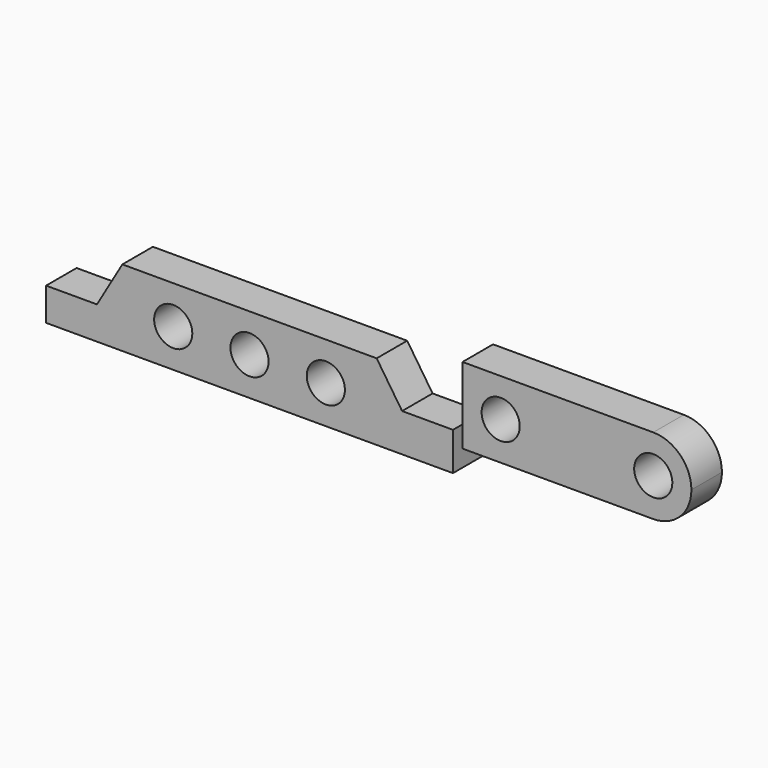
from build123d import *

# Parameters (mm, degrees)
F0_W     = 114.3
F0_H     = 38.1
F0_R     = 9.525
F1_DEPTH = 19.05
F2_R     = 19.04999
F3_R     = 9.525
F4_DEPTH = 19.05


# Not quite as in the source:
# - a fillet or chamfer is up to 0.001 mm smaller than in the source, because OpenCascade refuses the exact size


with BuildPart() as f1:
    # F0 (on Front) → F1 (new body)
    with BuildSketch(Plane.XZ):
        Rectangle(F0_W, F0_H)
        with Locations((-38.1, 0)):
            Circle(F0_R, mode=Mode.SUBTRACT)
        with Locations((38.1, 0)):
            Circle(F0_R, mode=Mode.SUBTRACT)
    extrude(amount=F1_DEPTH)

    # F2 (radius 19.05 in the source; OpenCascade refuses exactly that, so slightly less here)
    f2_edges = [f1.edges().sort_by_distance(p)[0] for p in [
        (57.15, -9.525, 19.05),
        (57.15, -9.525, -19.05),
    ]]
    fillet(f2_edges, radius=F2_R)


with BuildPart() as f4:
    # F3 (on Front) → F4 (new body)
    with BuildSketch(Plane.XZ):
        Polygon((-100.0284222552, 6.6953860101), (-227.0284222552, 6.6953860101), (-239.7284222552, -15.025992686), (-265.1284222552, -15.025992686), (-265.1284222552, -31.4046139899), (-61.9284222552, -31.4046139899), (-61.9284222552, -12.3546139899), (-87.3284222552, -12.3546139899), align=None)
        with Locations((-201.6284222552, -12.3546139899)):
            Circle(F3_R, mode=Mode.SUBTRACT)
        with Locations((-163.5284222552, -12.3546139899)):
            Circle(F3_R, mode=Mode.SUBTRACT)
        with Locations((-125.4284222552, -12.3546139899)):
            Circle(F3_R, mode=Mode.SUBTRACT)
    extrude(amount=F4_DEPTH)


solid = Compound([f1.part, f4.part])
